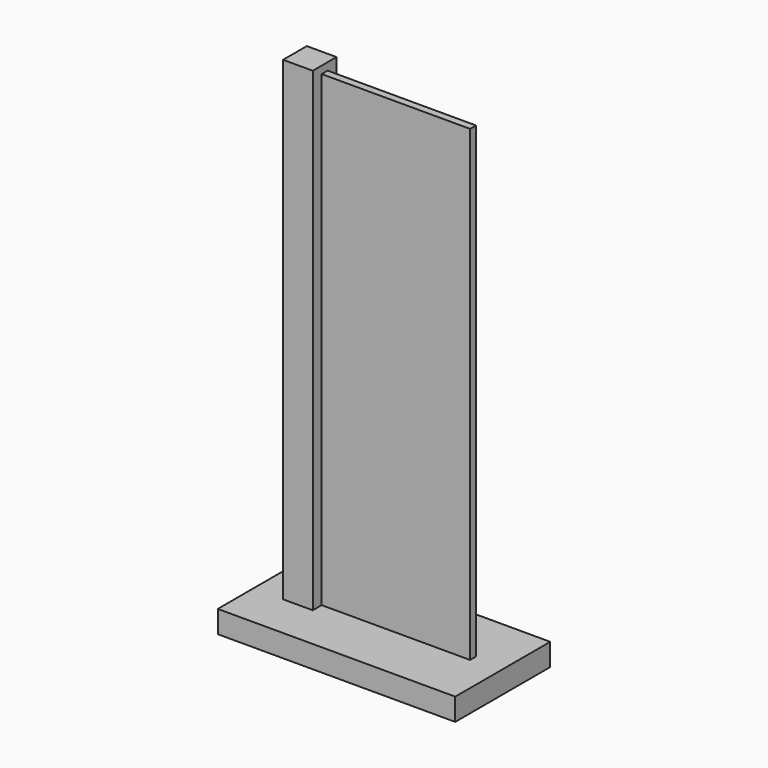
from build123d import *

# Parameters (mm, degrees)
F0_W     = 203.2
F0_H     = 101.6
F0_W_2   = 127
F0_H_2   = 6.35
F1_DEPTH = 19.05
F2_DEPTH = 406.4
F0_W_3   = 7.0298084438
F3_DEPTH = 400.05
F4_W     = 7.0298084438
F4_H     = 6.35
F5_DEPTH = 6.35


with BuildPart() as f1:
    # F0 (on Top) → F1 (new body)
    with BuildSketch(Plane.XY):
        Rectangle(F0_W, F0_H)
        Polygon((-76.2, 12.7), (-50.8, 12.7), (-50.8, 3.175), (76.2, 3.175), (76.2, -3.175), (-50.8, -3.175), (-50.8, -12.7), (-76.2, -12.7), align=None, mode=Mode.SUBTRACT)
        Polygon((-50.8, 3.175), (-50.8, 12.7), (-76.2, 12.7), (-76.2, -12.7), (-50.8, -12.7), (-50.8, -3.175), (-57.8298084438, -3.175), (-57.8298084438, 3.175), align=None)
        with Locations((12.7, 0)):
            Rectangle(F0_W_2, F0_H_2)
    extrude(amount=-F1_DEPTH)


with BuildPart() as f2:
    # F0 (on Top) → F2 (new body)
    with BuildSketch(Plane.XY):
        Polygon((-50.8, 3.175), (-50.8, 12.7), (-76.2, 12.7), (-76.2, -12.7), (-50.8, -12.7), (-50.8, -3.175), (-57.8298084438, -3.175), (-57.8298084438, 3.175), align=None)
    extrude(amount=F2_DEPTH)

    # F4 (on face) → F5 (join)
    with BuildSketch(Plane.XY.offset(406.4)):
        Polygon((-57.8298084438, -3.175), (-57.8298084438, 3.175), (-50.8, 3.175), (-50.8, 12.7), (-76.2, 12.7), (-76.2, -12.7), (-50.8, -12.7), (-50.8, -3.175), align=None)
        with Locations((-54.3149042219, 0)):
            Rectangle(F4_W, F4_H)
    extrude(amount=-F5_DEPTH)


with BuildPart() as f3:
    # F0 (on Top) → F3 (new body)
    with BuildSketch(Plane.XY):
        with Locations((12.7, 0)):
            Rectangle(F0_W_2, F0_H_2)
        with Locations((-54.3149042219, 0)):
            Rectangle(F0_W_3, F0_H_2)
    extrude(amount=F3_DEPTH)


solid = Compound([f1.part, f2.part, f3.part])
